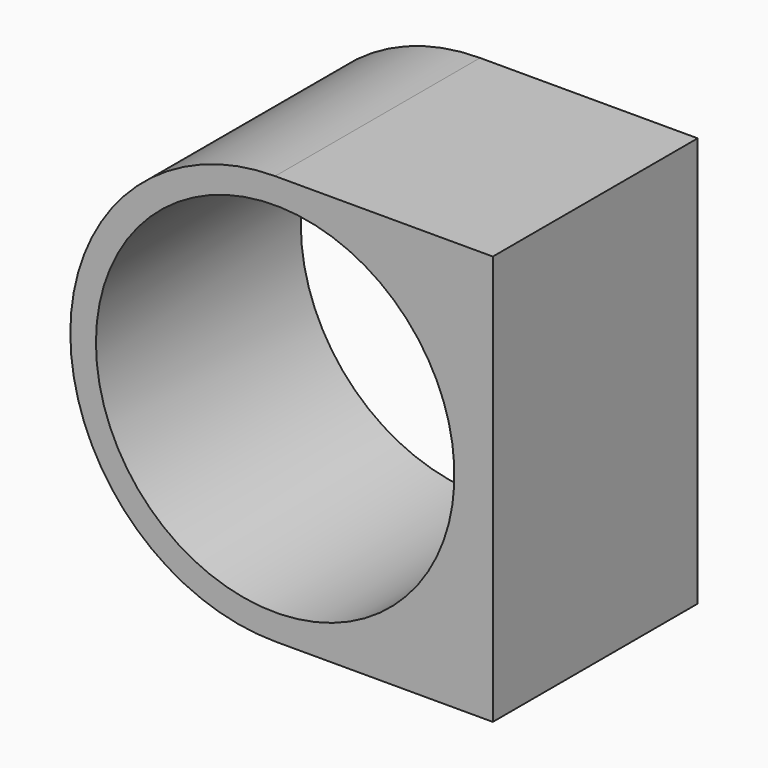
from build123d import *

# Parameters (mm, degrees)
F0_R      = 16
F0_R_2    = 10.5
F1_DEPTH  = 20
F2_R      = 12.5
F3_DEPTH  = 15
F4_DEPTH  = 15.001
F5_R      = 14
F6_DEPTH  = 15
F8_W      = 20
F8_H      = 16
F9_DEPTH  = 2
F11_DEPTH = 20
F14_DEPTH = 20
F15_DEPTH = 5.001


with BuildPart() as f1:
    # F0 (on Front) → F1 (new body)
    with BuildSketch(Plane.XZ):
        Circle(F0_R)
        Circle(F0_R_2, mode=Mode.SUBTRACT)
    extrude(amount=F1_DEPTH)

    # F2 (on face) → F3 (join)
    with BuildSketch(Plane.XZ.offset(20)):
        Circle(F2_R)
    extrude(amount=-F3_DEPTH)

    # F4 (cut, through all): a face of the model
    f4_faces = [f1.faces().sort_by_distance(p)[0] for p in [
        (0, -5, 0),
    ]]
    extrude(f4_faces, amount=-F4_DEPTH, mode=Mode.SUBTRACT)

    # F5 (on face) → F6 (cut)
    with BuildSketch(Plane(origin=(0, 0, 0), x_dir=(-1, 0, 0), z_dir=(0, 1, 0))):
        Circle(F5_R)
    extrude(amount=-F6_DEPTH, mode=Mode.SUBTRACT)

    # F8 (on offset) → F9 (join)
    with BuildSketch(Plane.YZ.offset(15)):
        with Locations((-10, -8)):
            Rectangle(F8_W, F8_H)
        with Locations((-10, 8)):
            Rectangle(F8_W, F8_H)
    extrude(amount=F9_DEPTH)

    # F10 (on face) → F11 (join)
    with BuildSketch(Plane.XZ.offset(20)):
        with BuildLine():
            Line((15, 16), (0, 16))
            ThreePointArc((0, 16), (9.1355287257, 13.1355287257), (15, 5.5677643628))
            Line((15, 5.5677643628), (15, 16))
        make_face()
    extrude(amount=-F11_DEPTH)

    # F13 (on face) → F14 (join)
    with BuildSketch(Plane.XZ.offset(20)):
        with BuildLine():
            Line((0, -16), (15, -16))
            Line((15, -16), (15, -5.5677643628))
            ThreePointArc((15, -5.5677643628), (9.1355287257, -13.1355287257), (0, -16))
        make_face()
    extrude(amount=-F14_DEPTH)

    # F15 (cut, through all): a face of the model
    f15_faces = [f1.faces().sort_by_distance(p)[0] for p in [
        (13.6040202025, -15, 0),
    ]]
    extrude(f15_faces, amount=-F15_DEPTH, mode=Mode.SUBTRACT)


solid = f1.part
